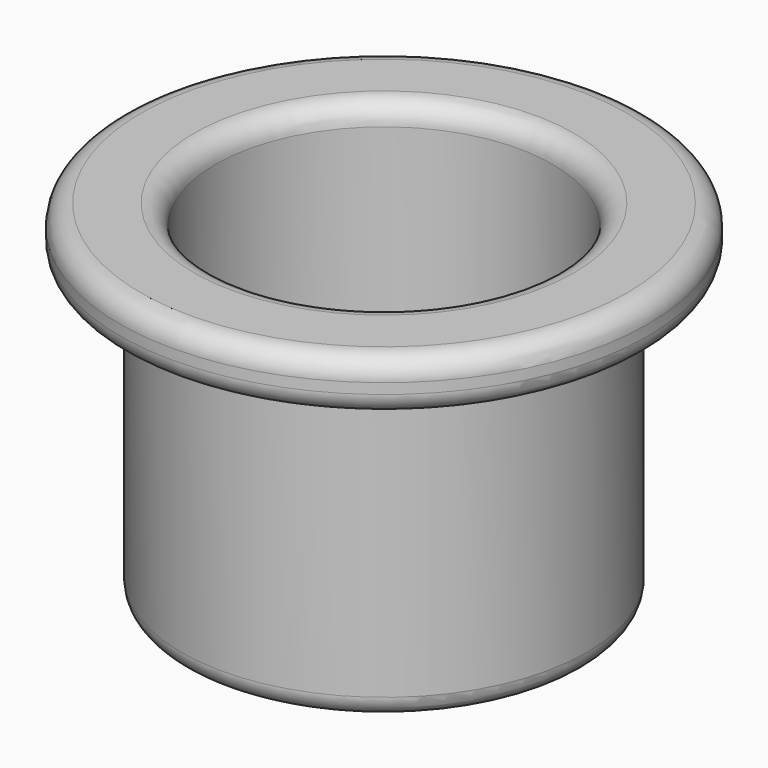
from build123d import *

# Parameters (mm, degrees)
F0_R     = 7.8105
F0_R_2   = 6.5
F1_DEPTH = 11.43
F2_R     = 10.16
F2_R_2   = 6.5
F3_DEPTH = 2
F4_R     = 0.8


# Not quite as in the source:
# - a fillet or chamfer that OpenCascade refuses, or shapes differently, is made with other operations: its cross-section is extruded or revolved along the edge and cut away or added


with BuildPart() as f1:
    # F0 (on Top) → F1 (new body)
    with BuildSketch(Plane.XY):
        Circle(F0_R)
        Circle(F0_R_2, mode=Mode.SUBTRACT)
    extrude(amount=F1_DEPTH)

    # F2 (on face) → F3 (join)
    with BuildSketch(Plane.XY.offset(11.43)):
        Circle(F2_R)
        Circle(F2_R_2, mode=Mode.SUBTRACT)
    extrude(amount=F3_DEPTH)

    # F4
    f4_edges = [f1.edges().sort_by_distance(p)[0] for p in [
        (-6.5, 0, 13.43),
        (-6.5, 0, 0),
        (-7.8105, 0, 11.43),
        (-10.16, 0, 13.43),
    ]]
    fillet(f4_edges, radius=F4_R)

    # F5: fillet of radius 0.8 on 2 edges, made by hand

    # F5_s1 → F5_t2 (revolve, cut)
    with BuildSketch(Plane.XZ):
        with BuildLine():
            ThreePointArc((7.8105, 0.7457813017), (7.6706514978, 0.2938963606), (7.3, 0))
            Line((7.3, 0), (7.8105, 0))
            Line((7.8105, 0), (7.8105, 0.7457813017))
        make_face()
    revolve(axis=Axis((0, 0, 0), (0, 0, 1)), mode=Mode.SUBTRACT)

    # F5_s3 → F5_t4 (revolve, cut)
    with BuildSketch(Plane.XZ):
        with BuildLine():
            ThreePointArc((9.36, 11.43), (9.9256854249, 11.6643145751), (10.16, 12.23))
            Line((10.16, 12.23), (10.16, 11.43))
            Line((10.16, 11.43), (9.36, 11.43))
        make_face()
    revolve(axis=Axis((0, 0, 11.43), (0, 0, 1)), mode=Mode.SUBTRACT)


solid = f1.part
